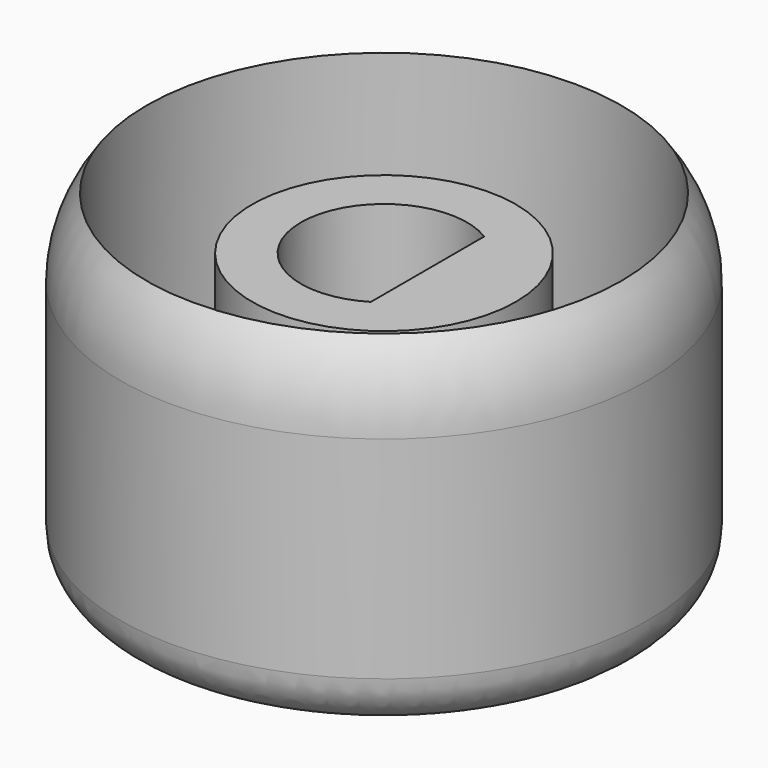
from build123d import *

# Parameters (mm, degrees)
F0_R     = 10
F0_R_2   = 5
F1_DEPTH = 4
F2_R     = 10
F2_R_2   = 9
F3_DEPTH = 12
F5_R     = 10
F6_DEPTH = 1
F7_R     = 2
F8_DEPTH = 10


# Not quite as in the source:
# - a fillet or chamfer that OpenCascade refuses, or shapes differently, is made with other operations: its cross-section is extruded or revolved along the edge and cut away or added


with BuildPart() as f1:
    # F0 (on Top) → F1 (new body)
    with BuildSketch(Plane.XY):
        Circle(F0_R)
        Circle(F0_R_2, mode=Mode.SUBTRACT)
    extrude(amount=F1_DEPTH)

    # F2 (on Top) → F3 (join)
    with BuildSketch(Plane.XY):
        Circle(F2_R)
        Circle(F2_R_2, mode=Mode.SUBTRACT)
    extrude(amount=F3_DEPTH)

    # F4: fillet of radius 5 on 1 edges, made by hand

    # F4_s1 → F4_t2 (revolve, cut)
    with BuildSketch(Plane.XZ):
        with BuildLine():
            ThreePointArc((10, 9), (9.7434164903, 10.5811388301), (9, 12))
            Line((9, 12), (10, 12))
            Line((10, 12), (10, 9))
        make_face()
    revolve(axis=Axis((0, 0, 12), (0, 0, 1)), mode=Mode.SUBTRACT)

    # F5 (on face) → F6 (join)
    with BuildSketch(Plane.XY):
        Circle(F5_R)
    extrude(amount=-F6_DEPTH)

    # F7
    f7_edges = [f1.edges().sort_by_distance(p)[0] for p in [
        (-10, 0, -1),
    ]]
    fillet(f7_edges, radius=F7_R)

    # F0 (on Top) → F8 (join)
    with BuildSketch(Plane.XY):
        Circle(F0_R_2)
        with BuildLine():
            ThreePointArc((1.65, -2.683281573), (-3.15, 0), (1.65, 2.683281573))
            Line((1.65, 2.683281573), (1.65, -2.683281573))
        make_face(mode=Mode.SUBTRACT)
    extrude(amount=F8_DEPTH)


solid = f1.part
